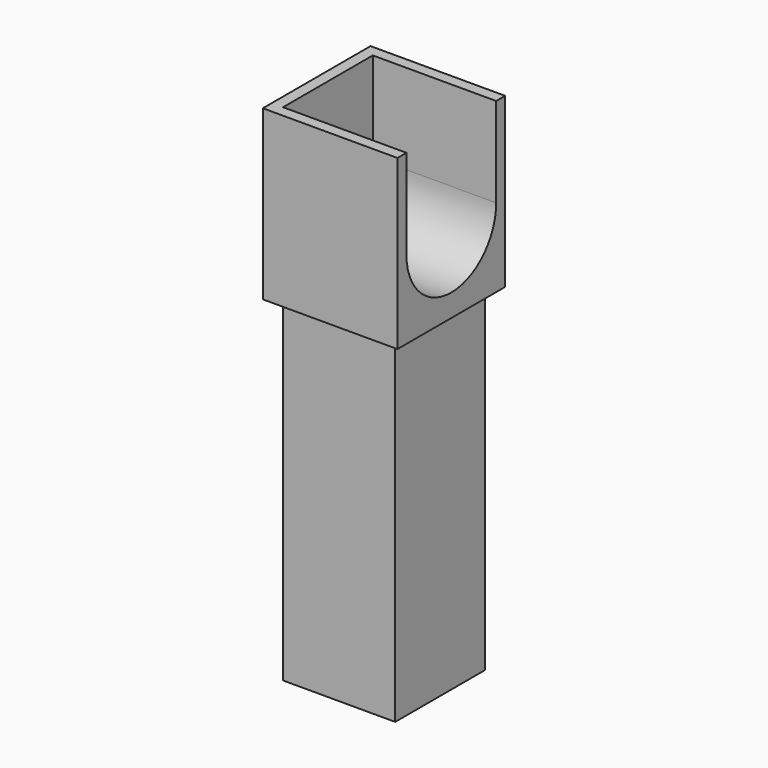
from build123d import *

# Parameters (mm, degrees)
F0_W      = 5
F0_H      = 22.5
F1_DEPTH  = 5
F2_R      = 0.6
F3_DEPTH  = 20
F4_W      = 5
F4_H      = 5
F5_DEPTH  = 5
F6_W      = 5
F6_H      = 5.0048647351
F7_DEPTH  = 0.5
F9_DEPTH  = 0.5
F11_DEPTH = 0.5
F13_DEPTH = 0.5
F15_DEPTH = 25
F16_DEPTH = 4
F17_DEPTH = 7.5
F19_DEPTH = 0.5


with BuildPart() as f1:
    # F0 (on Front) → F1 (new body)
    with BuildSketch(Plane.XZ):
        with Locations((-0.7514320314, 3.0499891839)):
            Rectangle(F0_W, F0_H)
    extrude(amount=F1_DEPTH)

    # F2 (on face) → F3 (cut)
    with BuildSketch(Plane(origin=(0, 0, -8.2000108161), x_dir=(1, 0, 0), z_dir=(0, 0, -1))):
        with Locations((-0.7514320314, 2.5)):
            Circle(F2_R)
    extrude(amount=-F3_DEPTH, mode=Mode.SUBTRACT)

    # F4 (on face) → F5 (join)
    with BuildSketch(Plane.XZ.offset(5)):
        with Locations((-0.7514320314, 16.7999891839)):
            Rectangle(F4_W, F4_H)
    extrude(amount=-F5_DEPTH)

    # F6 (on face) → F7 (join)
    with BuildSketch(Plane.YZ.offset(1.7485679686)):
        with Locations((-2.5, 16.7975568164)):
            Rectangle(F6_W, F6_H)
    extrude(amount=F7_DEPTH)

    # F8 (on face) → F9 (join)
    with BuildSketch(Plane(origin=(0, 0, 0), x_dir=(-1, 0, 0), z_dir=(0, 1, 0))):
        Polygon((-2.2485679686, 14.2951244488), (-1.7485679686, 14.2951244488), (3.2514320314, 14.2951244488), (3.2514320314, 19.2999891839), (-2.2485679686, 19.2999891839), align=None)
    extrude(amount=F9_DEPTH)

    # F10 (on face) → F11 (join)
    with BuildSketch(Plane.XZ.offset(5)):
        Polygon((-3.2514320314, 14.2951244488), (1.7485679686, 14.2951244488), (2.2485679686, 14.2951244488), (2.2485679686, 19.2999891839), (-3.2514320314, 19.2999891839), align=None)
    extrude(amount=F11_DEPTH)

    # F12 (on face) → F13 (join)
    with BuildSketch(Plane(origin=(-3.2514320314, 0, 0), x_dir=(0, -1, 0), z_dir=(-1, 0, 0))):
        Polygon((-0.5, 14.2951244488), (0, 14.2951244488), (5, 14.2951244488), (5.5, 14.2951244488), (5.5, 19.2999891839), (-0.5, 19.2999891839), align=None)
    extrude(amount=F13_DEPTH)

    # F14 (on face) → F15 (cut)
    with BuildSketch(Plane(origin=(-3.7514320314, 0, 0), x_dir=(0, -1, 0), z_dir=(-1, 0, 0))):
        with BuildLine():
            Line((-0.5, 17.7951244488), (0, 17.7951244488))
            ThreePointArc((0, 17.7951244488), (2.5, 15.2951244488), (5, 17.7951244488))
            Line((5, 17.7951244488), (5.5, 17.7951244488))
            Line((5.5, 17.7951244488), (5.5, 19.2999891839))
            Line((5.5, 19.2999891839), (-0.5, 19.2999891839))
            Line((-0.5, 19.2999891839), (-0.5, 17.7951244488))
        make_face()
    extrude(amount=-F15_DEPTH, mode=Mode.SUBTRACT)

    # F16 (add): faces of the model
    f16_faces = [f1.faces().sort_by_distance(p)[0] for p in [
        (-0.7514320314, -5.25, 17.7951244488),
        (-0.7514320314, 0.25, 17.7951244488),
    ]]
    extrude(f16_faces, amount=F16_DEPTH)

    # F17 (cut): a face of the model
    f17_faces = [f1.faces().sort_by_distance(p)[0] for p in [
        (-3.1807213533, -2.5, -8.2000108161),
    ]]
    extrude(f17_faces, amount=-F17_DEPTH, mode=Mode.SUBTRACT)

    # F18 (on face) → F19 (join)
    with BuildSketch(Plane(origin=(-3.7514320314, 0, 0), x_dir=(0, -1, 0), z_dir=(-1, 0, 0))):
        with BuildLine():
            Line((5, 21.7951244488), (0, 21.7951244488))
            Line((0, 21.7951244488), (0, 17.7951244488))
            ThreePointArc((0, 17.7951244488), (2.5, 15.2951244488), (5, 17.7951244488))
            Line((5, 17.7951244488), (5, 21.7951244488))
        make_face()
    extrude(amount=-F19_DEPTH)


solid = f1.part
